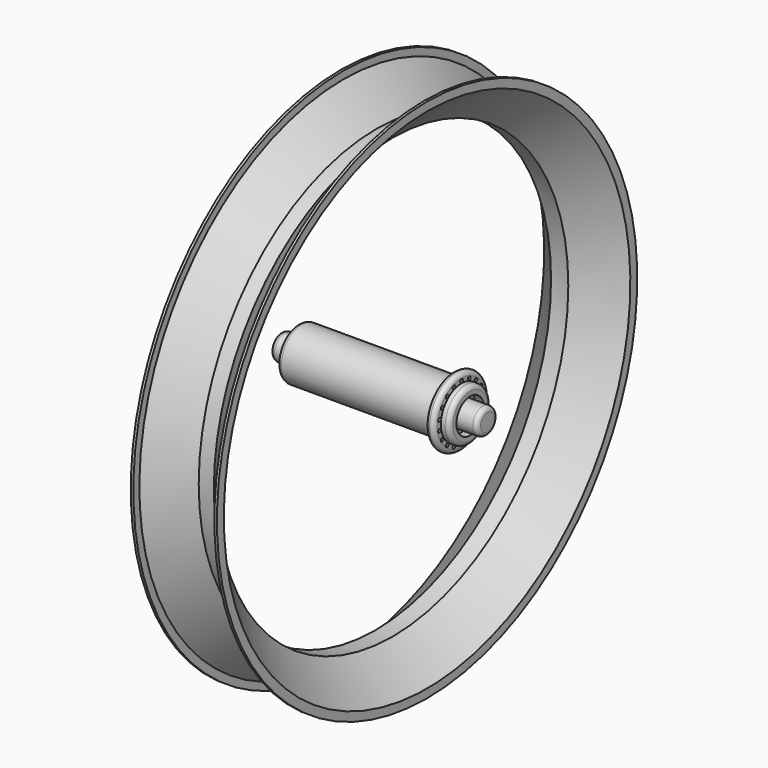
from build123d import *

# Parameters (mm, degrees)
F2_R     = 15
F3_DEPTH = 120
F4_R     = 20
F4_R_2   = 15
F5_DEPTH = 90
F4_R_3   = 30
F6_DEPTH = 100
F7_START = 80
F4_R_4   = 40
F7_DEPTH = 10
F8_R     = 4.99999
F8_2_R   = 4.99999
F9_D     = 4
F9_DEPTH = 16
F9_START = 80
F9_TIP   = 1.2017212381


# Not quite as in the source:
# - a fillet or chamfer is up to 0.001 mm smaller than in the source, because OpenCascade refuses the exact size


with BuildPart() as f1:
    # F0 (on Front) → F1 (revolve)
    with BuildSketch(Plane.XZ):
        Polygon((-50, 304.8), (-50, 294.8), (-10, 254.8), (0, 254.8), (10, 254.8), (50, 294.8), (50, 304.8), (46.9999983907, 304.8), (46.9999983907, 296.0426413537), (8.7573586463, 257.8000016093), (0, 257.8000016093), (-8.7573586463, 257.8000016093), (-46.9999983907, 296.0426413537), (-46.9999983907, 304.8), align=None)
    revolve(axis=Axis((62.5034868717, 0, 0), (1, 0, 0)))


with BuildPart() as f3:
    # F2 (on Right) → F3 (new body, symmetric)
    with BuildSketch(Plane.YZ):
        Circle(F2_R)
    extrude(amount=F3_DEPTH, both=True)

    # F4 (on Right) → F5 (join, symmetric)
    with BuildSketch(Plane.YZ):
        Circle(F4_R)
        Circle(F4_R_2, mode=Mode.SUBTRACT)
    extrude(amount=F5_DEPTH, both=True)

    # F4 (on Right) → F6 (join, symmetric)
    with BuildSketch(Plane.YZ):
        Circle(F4_R_3)
        Circle(F4_R, mode=Mode.SUBTRACT)
    extrude(amount=F6_DEPTH, both=True)

    # F8 (radius 5 in the source; OpenCascade refuses exactly that, so slightly less here)
    f8_edges = [f3.edges().sort_by_distance(p)[0] for p in [
        (120, -15, 0),
        (-120, -15, 0),
        (-100, -30, 0),
        (100, -30, 0),
    ]]
    fillet(f8_edges, radius=F8_R)


with BuildPart() as f7:
    # F4 (on Right) → F7 (new body)
    with BuildSketch(Plane.YZ.offset(F7_START)):
        Circle(F4_R_4)
        Circle(F4_R_3, mode=Mode.SUBTRACT)
    extrude(amount=F7_DEPTH)

    # F8#2 (radius 5 in the source; OpenCascade refuses exactly that, so slightly less here)
    f8_2_edges = [f7.edges().sort_by_distance(p)[0] for p in [
        (80, -40, 0),
        (90, -40, 0),
    ]]
    fillet(f8_2_edges, radius=F8_2_R)

    # F9
    # its depths count from where the whole tool has entered the part; down to there all is cleared
    with Locations(Plane(origin=(0, 0, 0), x_dir=(0, 1, 0), z_dir=(-1, 0, 0))):
        with Locations((0, -32.5), (11.1156546581, -30.5400101755), (20.8905973148, -24.8964444014), (28.145825623, -16.25), (32.0062519729, -5.6435657742), (32.0062519729, 5.6435657742), (28.145825623, 16.25), (20.8905973148, 24.8964444014), (11.1156546581, 30.5400101755), (0, 32.5), (-11.1156546581, 30.5400101755), (-20.8905973148, 24.8964444014), (-20.8905973148, 24.8964444014), (-28.145825623, 16.25), (-32.0062519729, 5.6435657742), (-32.0062519729, -5.6435657742), (-28.145825623, -16.25), (-20.8905973148, -24.8964444014), (-11.1156546581, -30.5400101755)):
            Hole(F9_D / 2, depth=F9_START)
    with Locations(Plane(origin=(0, 0, 0), x_dir=(0, 1, 0), z_dir=(-1, 0, 0)).offset(-F9_START)):
        with Locations((0, -32.5), (11.1156546581, -30.5400101755), (20.8905973148, -24.8964444014), (28.145825623, -16.25), (32.0062519729, -5.6435657742), (32.0062519729, 5.6435657742), (28.145825623, 16.25), (20.8905973148, 24.8964444014), (11.1156546581, 30.5400101755), (0, 32.5), (-11.1156546581, 30.5400101755), (-20.8905973148, 24.8964444014), (-20.8905973148, 24.8964444014), (-28.145825623, 16.25), (-32.0062519729, 5.6435657742), (-32.0062519729, -5.6435657742), (-28.145825623, -16.25), (-20.8905973148, -24.8964444014), (-11.1156546581, -30.5400101755)):
            Hole(F9_D / 2, depth=F9_DEPTH)
            with Locations((0, 0, -(F9_DEPTH + F9_TIP / 2))):  # 118° drill point
                Cone(0, F9_D / 2, F9_TIP, mode=Mode.SUBTRACT)


solid = Compound([f1.part, f3.part, f7.part])
